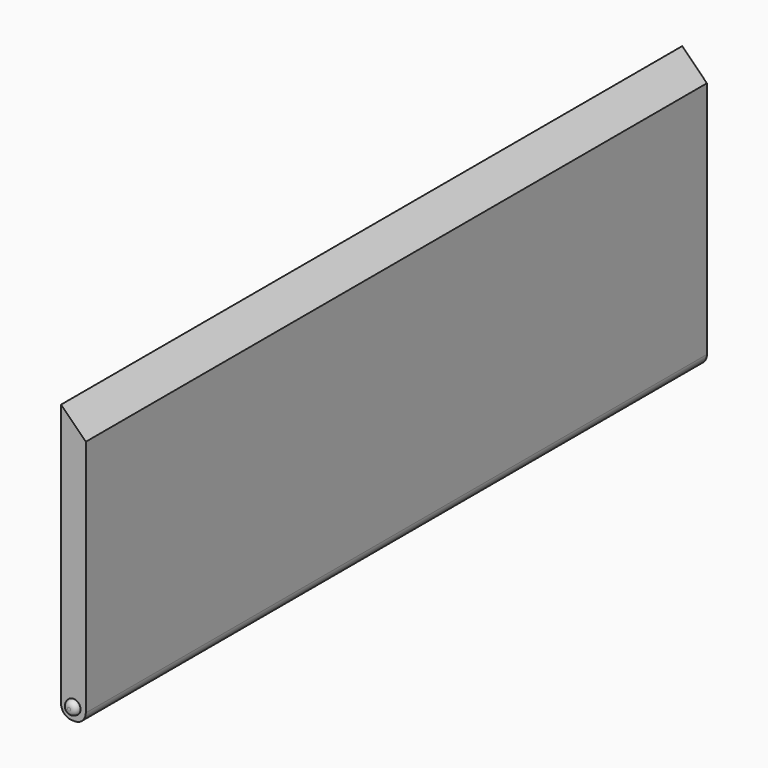
from build123d import *

# Parameters (mm, degrees)
F0_R     = 1.5
F1_DEPTH = 141.5
F0_R_2   = 1.3
F2_DEPTH = 141.5
F3_DEPTH = 142.5
F4_DEPTH = 2
F5_R     = 0.99999


# Not quite as in the source:
# - a fillet or chamfer is up to 0.001 mm smaller than in the source, because OpenCascade refuses the exact size


with BuildPart() as f1:
    # F0 (on Front) → F1 (new body)
    with BuildSketch(Plane.XZ):
        with BuildLine():
            Line((0.25, 46.7269286196), (-4.25, 51.2269286196))
            Line((-4.25, 51.2269286196), (-4.25, 3.2269286196))
            ThreePointArc((-4.25, 3.2269286196), (-3.6642135624, 1.8127150573), (-2.25, 1.2269286196))
            Line((-2.25, 1.2269286196), (-1.75, 1.2269286196))
            ThreePointArc((-1.75, 1.2269286196), (-0.3357864376, 1.8127150573), (0.25, 3.2269286196))
            Line((0.25, 3.2269286196), (0.25, 46.7269286196))
        make_face()
        with Locations((-2, 3.4769286196)):
            Circle(F0_R, mode=Mode.SUBTRACT)
    extrude(amount=F1_DEPTH)

    # F0 (on Front) → F2 (join)
    with BuildSketch(Plane.XZ):
        with Locations((-2, 3.4769286196)):
            Circle(F0_R)
        with Locations((-2, 3.4769286196)):
            Circle(F0_R_2, mode=Mode.SUBTRACT)
    extrude(amount=F2_DEPTH)

    # F0 (on Front) → F3 (join)
    with BuildSketch(Plane.XZ):
        with Locations((-2, 3.4769286196)):
            Circle(F0_R_2)
    extrude(amount=F3_DEPTH)

    # F0 (on Front) → F4 (cut)
    with BuildSketch(Plane.XZ):
        with Locations((-2, 3.4769286196)):
            Circle(F0_R)
        with Locations((-2, 3.4769286196)):
            Circle(F0_R_2, mode=Mode.SUBTRACT)
        with Locations((-2, 3.4769286196)):
            Circle(F0_R_2)
    extrude(amount=F4_DEPTH, mode=Mode.SUBTRACT)

    # F5 (radius 1 in the source; OpenCascade refuses exactly that, so slightly less here)
    f5_edges = [f1.edges().sort_by_distance(p)[0] for p in [
        (-3.3, -142.5, 3.476929),
    ]]
    fillet(f5_edges, radius=F5_R)


solid = f1.part
